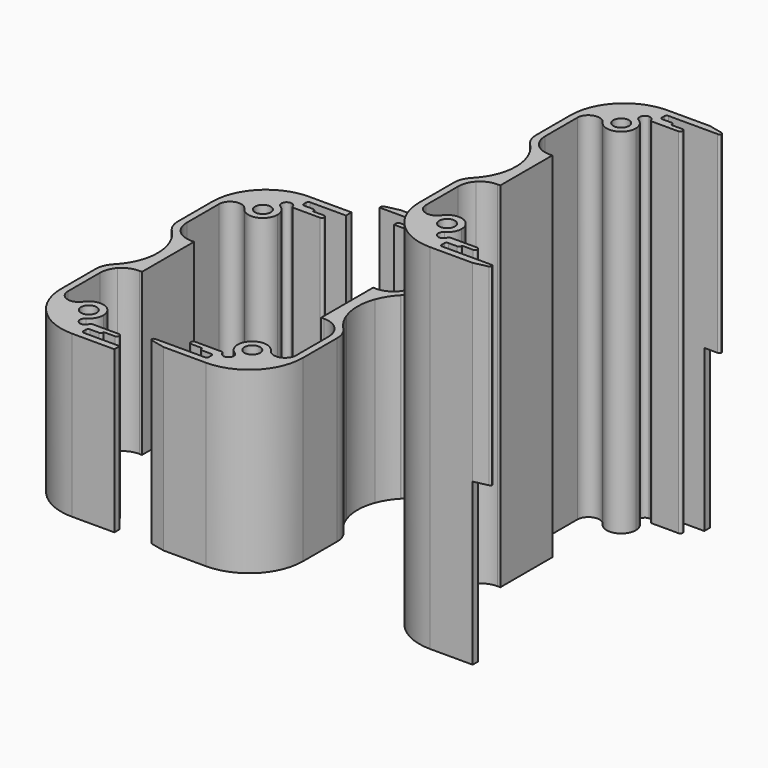
from build123d import *

# Parameters (mm, degrees)
F0_R          = 1.75
F0_W          = 4.8
F0_H          = 1.5477275198
F1_DEPTH      = 79
F2_DEPTH      = 40
F3_DEPTH      = 36
F4_T1_DEPTH   = 79
F4_T3_DEPTH   = 90.2941924891
F4_2_T1_DEPTH = 40
F4_2_T3_DEPTH = 51.2941924891
F4_3_T1_DEPTH = 36
F4_3_T3_DEPTH = 47.2941924891
F5_T1_DEPTH   = 79
F5_T3_DEPTH   = 81.0076197192
F5_T5_DEPTH   = 81.5
F5_T7_DEPTH   = 81.1160384943
F5_2_T1_DEPTH = 40
F5_2_T3_DEPTH = 42.0076197192
F5_2_T5_DEPTH = 42.5
F5_2_T7_DEPTH = 42.1160384943
F5_3_F1_R     = 0.5
F5_3_F2_R     = 0.4999
F5_3_F3_R     = 0.5
F5_3_F4_R     = 0.4999
F5_3_F5_R     = 0.5
F5_3_F6_R     = 0.5
F5_3_F7_R     = 0.5
F5_3_F8_R     = 0.5
F5_3_F9_R     = 0.5
F5_3_F10_R    = 0.5
F5_3_F11_R    = 0.5
F5_3_F12_R    = 0.5
F5_3_F13_R    = 0.5
F5_3_F14_R    = 0.5
F5_3_F15_R    = 0.5
F5_3_F16_R    = 0.5
F6_W          = 6
F6_H          = 66.2
F7_DEPTH      = 79.001
F8_W          = 6
F8_H          = 66.2
F9_DEPTH      = 36


# Not quite as in the source:
# - a fillet or chamfer that OpenCascade refuses, or shapes differently, is made with other operations: its cross-section is extruded or revolved along the edge and cut away or added
# - a fillet or chamfer is up to 0.001 mm smaller than in the source, because OpenCascade refuses the exact size


with BuildPart() as f1:
    # F0 (on Top) → F1 (new body)
    with BuildSketch(Plane.XY):
        with BuildLine():
            Line((-7, 11.0797111876), (-7, 9.2741576437))
            ThreePointArc((-7, 9.2741576437), (-6.2214566954, 8.6496058512), (-5.5, 7.9598994969))
            Line((-5.5, 7.9598994969), (-5.5, 10.0054984883))
            ThreePointArc((-5.5, 10.0054984883), (-6.2309192612, 10.5692486379), (-7, 11.0797111876))
        make_face()
        with BuildLine():
            ThreePointArc((-5.5, 21.1), (-2.7701351338, 28.1622234461), (4.0000000006, 31.5522724802))
            Line((4.0000000006, 31.5522724802), (4.0000000006, 33.0582607432))
            ThreePointArc((4.0000000006, 33.0582607432), (-3.8317608661, 29.2240384049), (-7, 21.1))
            Line((-7, 21.1), (-7, 11.0797111876))
            ThreePointArc((-7, 11.0797111876), (-6.2309192612, 10.5692486379), (-5.5, 10.0054984883))
            Line((-5.5, 10.0054984883), (-5.5, 21.1))
        make_face()
        with BuildLine():
            Line((-5.5, 10.0054984883), (-5.5, 7.9598994969))
            ThreePointArc((-5.5, 7.9598994969), (-4.0491111778, 6.0967341403), (-3.0093790725, 3.9764934301))
            Line((-3.0093790725, 3.9764934301), (-3.0093790725, 7.25))
            ThreePointArc((-3.0093790725, 7.25), (-4.1557714239, 8.7171586639), (-5.5, 10.0054984883))
        make_face()
        with BuildLine():
            Line((-3.0093790725, -3.9764934301), (-3.0093790725, -7.25))
            ThreePointArc((-3.0093790725, -7.25), (-1.3646055138, -3.7895862533), (-0.8, 0))
            ThreePointArc((-0.8, 0), (-1.3646055138, 3.7895862533), (-3.0093790725, 7.25))
            Line((-3.0093790725, 7.25), (-3.0093790725, 3.9764934301))
            ThreePointArc((-3.0093790725, 3.9764934301), (-2.4787337134, 2.0196360234), (-2.3, 0))
            ThreePointArc((-2.3, 0), (-2.4787337134, -2.0196360234), (-3.0093790725, -3.9764934301))
        make_face()
        with BuildLine():
            Line((-5.5, -7.9598994969), (-5.5, -10.0054984883))
            ThreePointArc((-5.5, -10.0054984883), (-4.1557714239, -8.7171586639), (-3.0093790725, -7.25))
            Line((-3.0093790725, -7.25), (-3.0093790725, -3.9764934301))
            ThreePointArc((-3.0093790725, -3.9764934301), (-4.0491111778, -6.0967341403), (-5.5, -7.9598994969))
        make_face()
        with BuildLine():
            Line((-7, -9.2741576437), (-7, -11.0797111876))
            ThreePointArc((-7, -11.0797111876), (-6.2309192612, -10.5692486379), (-5.5, -10.0054984883))
            Line((-5.5, -10.0054984883), (-5.5, -7.9598994969))
            ThreePointArc((-5.5, -7.9598994969), (-6.2214566954, -8.6496058512), (-7, -9.2741576437))
        make_face()
        with BuildLine():
            Line((5, -33.1), (6.0000000006, -33.1))
            Line((6.0000000006, -33.1), (6.0000000006, -31.6))
            Line((6.0000000006, -31.6), (5, -31.6))
            ThreePointArc((5, -31.6), (4.4994308452, -31.5880613328), (4.0000000006, -31.5522724802))
            ThreePointArc((4.0000000006, -31.5522724802), (-2.7701351338, -28.1622234461), (-5.5, -21.1))
            Line((-5.5, -21.1), (-5.5, -10.0054984883))
            ThreePointArc((-5.5, -10.0054984883), (-6.2309192612, -10.5692486379), (-7, -11.0797111876))
            Line((-7, -11.0797111876), (-7, -21.1))
            ThreePointArc((-7, -21.1), (-3.4852813742, -29.5852813742), (5, -33.1))
        make_face()
        with BuildLine():
            ThreePointArc((-5.5, -21.1), (-2.7701351338, -28.1622234461), (4.0000000006, -31.5522724802))
            Line((4.0000000006, -31.5522724802), (4.0000000006, -29.2661634937))
            ThreePointArc((4.0000000006, -29.2661634937), (2.875248939, -28.408013544), (3.4058490733, -27.0965449838))
            ThreePointArc((3.4058490733, -27.0965449838), (-0.6127011239, -26.5316234895), (-0.9475889999, -22.4874014267))
            ThreePointArc((-0.9475889999, -22.4874014267), (-3.7375818679, -23.4795655398), (-5.5, -21.1))
        make_face()
        with BuildLine():
            ThreePointArc((5, -24.3), (2.6974533631, -21.1911686883), (-0.9475889999, -22.4874014267))
            ThreePointArc((-0.9475889999, -22.4874014267), (-0.6127011239, -26.5316234895), (3.4058490733, -27.0965449838))
            ThreePointArc((3.4058490733, -27.0965449838), (4.5734738788, -25.9095015551), (5, -24.3))
        make_face()
        with Locations((1.75, -24.3)):
            Circle(F0_R, mode=Mode.SUBTRACT)
        with BuildLine():
            Line((5, -31.6), (6.0000000006, -31.6))
            Line((6.0000000006, -31.6), (6.0000000006, -29.9))
            Line((6.0000000006, -29.9), (9.0000000006, -29.9))
            Line((9.0000000006, -29.9), (9.0000000006, -29.2))
            Line((9.0000000006, -29.2), (12.0000000006, -29.2))
            Line((12.0000000006, -29.2), (12.0000000006, -28.1))
            Line((12.0000000006, -28.1), (5.1661634942, -28.1))
            ThreePointArc((5.1661634942, -28.1), (4.8246021149, -28.9246021143), (4.0000000006, -29.2661634937))
            Line((4.0000000006, -29.2661634937), (4.0000000006, -31.5522724802))
            ThreePointArc((4.0000000006, -31.5522724802), (4.4994308452, -31.5880613328), (5, -31.6))
        make_face()
        Polygon((6.0000000006, -33.1), (14.5, -33.1), (18, -32.3261362401), (18, -31.6), (6.0000000006, -31.6), align=None)
        with BuildLine():
            Line((4.0000000006, 29.2661634937), (4.0000000006, 31.5522724802))
            ThreePointArc((4.0000000006, 31.5522724802), (-2.7701351338, 28.1622234461), (-5.5, 21.1))
            ThreePointArc((-5.5, 21.1), (-3.7375818642, 23.4795655409), (-0.9475889956, 22.4874014203))
            ThreePointArc((-0.9475889956, 22.4874014203), (-0.612701148, 26.531623464), (3.4058490196, 27.0965450156))
            ThreePointArc((3.4058490196, 27.0965450156), (2.8752489472, 28.408013574), (4.0000000006, 29.2661634937))
        make_face()
        with BuildLine():
            ThreePointArc((3.4058490196, 27.0965450156), (-0.612701148, 26.531623464), (-0.9475889956, 22.4874014203))
            ThreePointArc((-0.9475889956, 22.4874014203), (2.6974533668, 21.1911686894), (5, 24.3))
            ThreePointArc((5, 24.3), (4.5734738633, 25.9095015822), (3.4058490196, 27.0965450156))
        make_face()
        with Locations((1.75, 24.3)):
            Circle(F0_R, mode=Mode.SUBTRACT)
        with BuildLine():
            Line((6.0000000006, 29.9), (6.0000000006, 31.5522724802))
            Line((6.0000000006, 31.5522724802), (4.0000000006, 31.5522724802))
            Line((4.0000000006, 31.5522724802), (4.0000000006, 29.2661634937))
            ThreePointArc((4.0000000006, 29.2661634937), (4.8246021149, 28.9246021143), (5.1661634942, 28.1))
            Line((5.1661634942, 28.1), (12.0000000006, 28.1))
            Line((12.0000000006, 28.1), (12.0000000006, 29.2))
            Line((12.0000000006, 29.2), (9.0000000006, 29.2))
            Line((9.0000000006, 29.2), (9.0000000006, 29.9))
            Line((9.0000000006, 29.9), (6.0000000006, 29.9))
        make_face()
        with Locations((8.4000000006, 32.3261362401)):
            Rectangle(F0_W, F0_H)
        Polygon((10.8000000006, 31.5522724802), (18, 31.5522724802), (18, 32.3261362401), (14.5, 33.1), (10.8000000006, 33.1), align=None)
        with BuildLine():
            Line((4.0000000006, 31.5522724802), (6.0000000006, 31.5522724802))
            Line((6.0000000006, 31.5522724802), (6.0000000006, 33.1))
            Line((6.0000000006, 33.1), (5, 33.1))
            ThreePointArc((5, 33.1), (4.4995646484, 33.0895606449), (4.0000000006, 33.0582607432))
            Line((4.0000000006, 33.0582607432), (4.0000000006, 31.5522724802))
        make_face()
        with BuildLine():
            ThreePointArc((-0.8, 0), (-1.3646055138, -3.7895862533), (-3.0093790725, -7.25))
            Line((-3.0093790725, -7.25), (0, -7.25))
            Line((0, -7.25), (0, 7.25))
            Line((0, 7.25), (-3.0093790725, 7.25))
            ThreePointArc((-3.0093790725, 7.25), (-1.3646055138, 3.7895862533), (-0.8, 0))
        make_face()
    extrude(amount=F1_DEPTH)

    # F4: fillet of radius 5 on 6 edges, made by hand

    # F4_s2 → F4_t1 (join)
    with BuildSketch(Plane.XY):
        with BuildLine():
            ThreePointArc((-5.5, -12.1288911282), (-5.1622002436, -10.3222675125), (-4.1944444444, -8.7597547037))
            ThreePointArc((-4.1944444444, -8.7597547037), (-4.8255808359, -9.405307048), (-5.5, -10.0054984883))
            Line((-5.5, -10.0054984883), (-5.5, -12.1288911282))
        make_face()
        with BuildLine():
            ThreePointArc((-4.2749457245, -8.8472222222), (-2.6097264456, -7.6666666667), (-0.6114633109, -7.25))
            Line((-0.6114633109, -7.25), (-3.0093790725, -7.25))
            ThreePointArc((-3.0093790725, -7.25), (-3.6108172828, -8.0734475632), (-4.2749457245, -8.8472222222))
        make_face()
        with BuildLine():
            ThreePointArc((-4.1944444444, 8.7597547037), (-5.1622002436, 10.3222675125), (-5.5, 12.1288911282))
            Line((-5.5, 12.1288911282), (-5.5, 10.0054984883))
            ThreePointArc((-5.5, 10.0054984883), (-4.8255808359, 9.405307048), (-4.1944444444, 8.7597547037))
        make_face()
        with BuildLine():
            ThreePointArc((-0.6114633109, 7.25), (-2.6097264456, 7.6666666667), (-4.2749457245, 8.8472222222))
            ThreePointArc((-4.2749457245, 8.8472222222), (-3.6108172828, 8.0734475632), (-3.0093790725, 7.25))
            Line((-3.0093790725, 7.25), (-0.6114633109, 7.25))
        make_face()
    extrude(amount=F4_T1_DEPTH)

    # F4_s4 → F4_t3 (cut)
    with BuildSketch(Plane.XY.offset(-5.6470962445)):
        with BuildLine():
            ThreePointArc((-5.5757575758, 8.0381488259), (-6.6302693161, 9.6460393162), (-7, 11.5329961415))
            Line((-7, 11.5329961415), (-7, 9.2741576437))
            ThreePointArc((-7, 9.2741576437), (-6.2625007758, 8.6853961018), (-5.5757575758, 8.0381488259))
        make_face()
        with BuildLine():
            ThreePointArc((-5.5757575758, -8.0381488259), (-6.6302693161, -9.6460393162), (-7, -11.5329961415))
            Line((-7, -11.5329961415), (-7, -9.2741576437))
            ThreePointArc((-7, -9.2741576437), (-6.2625007758, -8.6853961018), (-5.5757575758, -8.0381488259))
        make_face()
    extrude(amount=F4_T3_DEPTH, mode=Mode.SUBTRACT)

    # F5: fillet of radius 0.5 on 16 edges, made by hand

    # F5_s2 → F5_t1 (join)
    with BuildSketch(Plane.XY):
        with BuildLine():
            ThreePointArc((6.5000000006, -29.9), (6.14644661, -30.0464466094), (6.0000000006, -30.4))
            Line((6.0000000006, -30.4), (6.0000000006, -29.9))
            Line((6.0000000006, -29.9), (6.5000000006, -29.9))
        make_face()
        with BuildLine():
            ThreePointArc((6.0000000006, -31.1), (6.14644661, -31.4535533906), (6.5000000006, -31.6))
            Line((6.5000000006, -31.6), (6.0000000006, -31.6))
            Line((6.0000000006, -31.6), (6.0000000006, -31.1))
        make_face()
        with BuildLine():
            ThreePointArc((6.5000000006, 31.5522724802), (6.14644661, 31.4058258708), (6.0000000006, 31.0522724802))
            Line((6.0000000006, 31.0522724802), (6.0000000006, 31.5522724802))
            Line((6.0000000006, 31.5522724802), (6.5000000006, 31.5522724802))
        make_face()
        with BuildLine():
            ThreePointArc((6.0000000006, 30.4), (6.14644661, 30.0464466094), (6.5000000006, 29.9))
            Line((6.5000000006, 29.9), (6.0000000006, 29.9))
            Line((6.0000000006, 29.9), (6.0000000006, 30.4))
        make_face()
    extrude(amount=F5_T1_DEPTH)

    # F5_s4 → F5_t3 (cut)
    with BuildSketch(Plane.XY.offset(-1.0038098596)):
        with BuildLine():
            ThreePointArc((18, -31.9246122963), (17.8898541073, -32.2376838137), (17.6079449, -32.4128211641))
            Line((17.6079449, -32.4128211641), (18, -32.3261362401))
            Line((18, -32.3261362401), (18, -31.9246122963))
        make_face()
        with BuildLine():
            ThreePointArc((17.6079449, 32.4128211641), (17.8898541073, 32.2376838137), (18, 31.9246122963))
            Line((18, 31.9246122963), (18, 32.3261362401))
            Line((18, 32.3261362401), (17.6079449, 32.4128211641))
        make_face()
    extrude(amount=F5_T3_DEPTH, mode=Mode.SUBTRACT)

    # F5_s6 → F5_t5 (cut)
    with BuildSketch(Plane.XY.offset(-1.25)):
        with BuildLine():
            ThreePointArc((17.5, -31.6), (17.8535533906, -31.7464466094), (18, -32.1))
            Line((18, -32.1), (18, -31.6))
            Line((18, -31.6), (17.5, -31.6))
        make_face()
        with BuildLine():
            ThreePointArc((9.0000000006, -29.4), (8.8535533912, -29.7535533906), (8.5000000006, -29.9))
            Line((8.5000000006, -29.9), (9.0000000006, -29.9))
            Line((9.0000000006, -29.9), (9.0000000006, -29.4))
        make_face()
        with BuildLine():
            ThreePointArc((12.0000000006, -28.7), (11.8535533912, -29.0535533906), (11.5000000006, -29.2))
            Line((11.5000000006, -29.2), (12.0000000006, -29.2))
            Line((12.0000000006, -29.2), (12.0000000006, -28.7))
        make_face()
        with BuildLine():
            ThreePointArc((11.5000000006, -28.1), (11.8535533912, -28.2464466094), (12.0000000006, -28.6))
            Line((12.0000000006, -28.6), (12.0000000006, -28.1))
            Line((12.0000000006, -28.1), (11.5000000006, -28.1))
        make_face()
        with BuildLine():
            ThreePointArc((18, 32.0522724802), (17.8535533906, 31.6987190896), (17.5, 31.5522724802))
            Line((17.5, 31.5522724802), (18, 31.5522724802))
            Line((18, 31.5522724802), (18, 32.0522724802))
        make_face()
        with BuildLine():
            ThreePointArc((8.5000000006, 29.9), (8.8535533912, 29.7535533906), (9.0000000006, 29.4))
            Line((9.0000000006, 29.4), (9.0000000006, 29.9))
            Line((9.0000000006, 29.9), (8.5000000006, 29.9))
        make_face()
        with BuildLine():
            ThreePointArc((12.0000000006, 28.6), (11.8535533912, 28.2464466094), (11.5000000006, 28.1))
            Line((11.5000000006, 28.1), (12.0000000006, 28.1))
            Line((12.0000000006, 28.1), (12.0000000006, 28.6))
        make_face()
        with BuildLine():
            ThreePointArc((11.5000000006, 29.2), (11.8535533912, 29.0535533906), (12.0000000006, 28.7))
            Line((12.0000000006, 28.7), (12.0000000006, 29.2))
            Line((12.0000000006, 29.2), (11.5000000006, 29.2))
        make_face()
    extrude(amount=F5_T5_DEPTH, mode=Mode.SUBTRACT)

    # F5_s8 → F5_t7 (cut)
    with BuildSketch(Plane.XY.offset(-1.0580192471)):
        with BuildLine():
            ThreePointArc((5.1124158407, -28.4499547008), (5.293586347, -28.1968730661), (5.5893711931, -28.1))
            Line((5.5893711931, -28.1), (5.1661634942, -28.1))
            ThreePointArc((5.1661634942, -28.1), (5.1526482636, -28.277029025), (5.1124158407, -28.4499547008))
        make_face()
        with BuildLine():
            ThreePointArc((5.5893711931, 28.1), (5.293586347, 28.1968730661), (5.1124158407, 28.4499547008))
            ThreePointArc((5.1124158407, 28.4499547008), (5.1526482636, 28.277029025), (5.1661634942, 28.1))
            Line((5.1661634942, 28.1), (5.5893711931, 28.1))
        make_face()
    extrude(amount=F5_T7_DEPTH, mode=Mode.SUBTRACT)

    # F8 (on face) → F9 (cut)
    with BuildSketch(Plane(origin=(0, 0, 0), x_dir=(1, 0, 0), z_dir=(0, 0, -1))):
        with Locations((17.5, 0)):
            Rectangle(F8_W, F8_H)
    extrude(amount=-F9_DEPTH, mode=Mode.SUBTRACT)


with BuildPart() as f2:
    # F0 (on Top) → F2 (new body)
    with BuildSketch(Plane.XY):
        with BuildLine():
            ThreePointArc((-34.5, 10.0054984883), (-33.7690807388, 10.5692486379), (-33, 11.0797111876))
            Line((-33, 11.0797111876), (-33, 21.1))
            ThreePointArc((-33, 21.1), (-36.1682391339, 29.2240384049), (-44.0000000006, 33.0582607432))
            Line((-44.0000000006, 33.0582607432), (-44.0000000006, 31.5522724802))
            ThreePointArc((-44.0000000006, 31.5522724802), (-37.2298648662, 28.1622234461), (-34.5, 21.1))
            Line((-34.5, 21.1), (-34.5, 10.0054984883))
        make_face()
        Polygon((-54.5, -33.1), (-46.0000000006, -33.1), (-46.0000000006, -31.6), (-58, -31.6), (-58, -32.3261362401), align=None)
        with BuildLine():
            Line((-33, -21.1), (-33, -11.0797111876))
            ThreePointArc((-33, -11.0797111876), (-33.7690807388, -10.5692486379), (-34.5, -10.0054984883))
            Line((-34.5, -10.0054984883), (-34.5, -21.1))
            ThreePointArc((-34.5, -21.1), (-37.2298648662, -28.1622234461), (-44.0000000006, -31.5522724802))
            ThreePointArc((-44.0000000006, -31.5522724802), (-44.4994308452, -31.5880613328), (-45, -31.6))
            Line((-45, -31.6), (-46.0000000006, -31.6))
            Line((-46.0000000006, -31.6), (-46.0000000006, -33.1))
            Line((-46.0000000006, -33.1), (-45, -33.1))
            ThreePointArc((-45, -33.1), (-36.5147186258, -29.5852813742), (-33, -21.1))
        make_face()
        with BuildLine():
            ThreePointArc((-45, -31.6), (-44.4994308452, -31.5880613328), (-44.0000000006, -31.5522724802))
            Line((-44.0000000006, -31.5522724802), (-44.0000000006, -29.2661634937))
            ThreePointArc((-44.0000000006, -29.2661634937), (-44.8246021149, -28.9246021143), (-45.1661634942, -28.1))
            Line((-45.1661634942, -28.1), (-52.0000000006, -28.1))
            Line((-52.0000000006, -28.1), (-52.0000000006, -29.2))
            Line((-52.0000000006, -29.2), (-49.0000000006, -29.2))
            Line((-49.0000000006, -29.2), (-49.0000000006, -29.9))
            Line((-49.0000000006, -29.9), (-46.0000000006, -29.9))
            Line((-46.0000000006, -29.9), (-46.0000000006, -31.6))
            Line((-46.0000000006, -31.6), (-45, -31.6))
        make_face()
        with BuildLine():
            ThreePointArc((-44.0000000006, -31.5522724802), (-37.2298648662, -28.1622234461), (-34.5, -21.1))
            ThreePointArc((-34.5, -21.1), (-36.2624181353, -23.4795655408), (-39.0524110039, -22.4874014212))
            ThreePointArc((-39.0524110039, -22.4874014212), (-38.6411686893, -23.3525466337), (-38.5, -24.3))
            ThreePointArc((-38.5, -24.3), (-40.1404982423, -27.1234737633), (-43.4058486719, -27.0965452215))
            ThreePointArc((-43.4058486719, -27.0965452215), (-42.9868823166, -27.5224795654), (-42.8338365069, -28.1))
            ThreePointArc((-42.8338365069, -28.1), (-43.1753978863, -28.9246021143), (-44.0000000006, -29.2661634937))
            Line((-44.0000000006, -29.2661634937), (-44.0000000006, -31.5522724802))
        make_face()
        with BuildLine():
            ThreePointArc((-38.5, -24.3), (-38.6411686893, -23.3525466337), (-39.0524110039, -22.4874014212))
            ThreePointArc((-39.0524110039, -22.4874014212), (-44.1127012864, -22.0683766825), (-43.4058486719, -27.0965452215))
            ThreePointArc((-43.4058486719, -27.0965452215), (-40.1404982423, -27.1234737633), (-38.5, -24.3))
        make_face()
        with Locations((-41.75, -24.3)):
            Circle(F0_R, mode=Mode.SUBTRACT)
        with BuildLine():
            ThreePointArc((-34.5, -10.0054984883), (-33.7690807388, -10.5692486379), (-33, -11.0797111876))
            Line((-33, -11.0797111876), (-33, -9.2741576437))
            ThreePointArc((-33, -9.2741576437), (-33.7785433046, -8.6496058512), (-34.5, -7.9598994969))
            Line((-34.5, -7.9598994969), (-34.5, -10.0054984883))
        make_face()
        with BuildLine():
            ThreePointArc((-36.9906209275, -7.25), (-35.8442285761, -8.7171586639), (-34.5, -10.0054984883))
            Line((-34.5, -10.0054984883), (-34.5, -7.9598994969))
            ThreePointArc((-34.5, -7.9598994969), (-35.9508888222, -6.0967341403), (-36.9906209275, -3.9764934301))
            Line((-36.9906209275, -3.9764934301), (-36.9906209275, -7.25))
        make_face()
        with BuildLine():
            Line((-40, -7.25), (-36.9906209275, -7.25))
            ThreePointArc((-36.9906209275, -7.25), (-39.2, 0), (-36.9906209275, 7.25))
            Line((-36.9906209275, 7.25), (-40, 7.25))
            Line((-40, 7.25), (-40, -7.25))
        make_face()
        with BuildLine():
            ThreePointArc((-36.9906209275, 7.25), (-39.2, 0), (-36.9906209275, -7.25))
            Line((-36.9906209275, -7.25), (-36.9906209275, -3.9764934301))
            ThreePointArc((-36.9906209275, -3.9764934301), (-37.7, 0), (-36.9906209275, 3.9764934301))
            Line((-36.9906209275, 3.9764934301), (-36.9906209275, 7.25))
        make_face()
        with BuildLine():
            ThreePointArc((-36.9906209275, 3.9764934301), (-35.9508888222, 6.0967341403), (-34.5, 7.9598994969))
            Line((-34.5, 7.9598994969), (-34.5, 10.0054984883))
            ThreePointArc((-34.5, 10.0054984883), (-35.8442285761, 8.7171586639), (-36.9906209275, 7.25))
            Line((-36.9906209275, 7.25), (-36.9906209275, 3.9764934301))
        make_face()
        with BuildLine():
            ThreePointArc((-34.5, 7.9598994969), (-33.7785433046, 8.6496058512), (-33, 9.2741576437))
            Line((-33, 9.2741576437), (-33, 11.0797111876))
            ThreePointArc((-33, 11.0797111876), (-33.7690807388, 10.5692486379), (-34.5, 10.0054984883))
            Line((-34.5, 10.0054984883), (-34.5, 7.9598994969))
        make_face()
        with BuildLine():
            ThreePointArc((-39.0524110298, 22.4874013826), (-36.2624181576, 23.4795655476), (-34.5, 21.1))
            ThreePointArc((-34.5, 21.1), (-37.2298648662, 28.1622234461), (-44.0000000006, 31.5522724802))
            Line((-44.0000000006, 31.5522724802), (-44.0000000006, 29.2661634937))
            ThreePointArc((-44.0000000006, 29.2661634937), (-43.1753978863, 28.9246021143), (-42.8338365069, 28.1))
            ThreePointArc((-42.8338365069, 28.1), (-42.9868823175, 27.5224795638), (-43.4058486751, 27.0965452196))
            ThreePointArc((-43.4058486751, 27.0965452196), (-40.1404982439, 27.1234737642), (-38.5, 24.3))
            ThreePointArc((-38.5, 24.3), (-38.641168696, 23.3525466115), (-39.0524110298, 22.4874013826))
        make_face()
        with BuildLine():
            ThreePointArc((-43.4058486751, 27.0965452196), (-44.1127013011, 22.068376698), (-39.0524110298, 22.4874013826))
            ThreePointArc((-39.0524110298, 22.4874013826), (-38.641168696, 23.3525466115), (-38.5, 24.3))
            ThreePointArc((-38.5, 24.3), (-40.1404982439, 27.1234737642), (-43.4058486751, 27.0965452196))
        make_face()
        with Locations((-41.75, 24.3)):
            Circle(F0_R, mode=Mode.SUBTRACT)
        with BuildLine():
            Line((-44.0000000006, 29.2661634937), (-44.0000000006, 31.5522724802))
            Line((-44.0000000006, 31.5522724802), (-46.0000000006, 31.5522724802))
            Line((-46.0000000006, 31.5522724802), (-46.0000000006, 29.9))
            Line((-46.0000000006, 29.9), (-49.0000000006, 29.9))
            Line((-49.0000000006, 29.9), (-49.0000000006, 29.2))
            Line((-49.0000000006, 29.2), (-52.0000000006, 29.2))
            Line((-52.0000000006, 29.2), (-52.0000000006, 28.1))
            Line((-52.0000000006, 28.1), (-45.1661634942, 28.1))
            ThreePointArc((-45.1661634942, 28.1), (-44.8246021149, 28.9246021143), (-44.0000000006, 29.2661634937))
        make_face()
        with Locations((-48.4000000006, 32.3261362401)):
            Rectangle(F0_W, F0_H)
        Polygon((-58, 32.3261362401), (-58, 31.5522724802), (-50.8000000006, 31.5522724802), (-50.8000000006, 33.1), (-54.5, 33.1), align=None)
        with BuildLine():
            Line((-44.0000000006, 31.5522724802), (-44.0000000006, 33.0582607432))
            ThreePointArc((-44.0000000006, 33.0582607432), (-44.4995646484, 33.0895606449), (-45, 33.1))
            Line((-45, 33.1), (-46.0000000006, 33.1))
            Line((-46.0000000006, 33.1), (-46.0000000006, 31.5522724802))
            Line((-46.0000000006, 31.5522724802), (-44.0000000006, 31.5522724802))
        make_face()
    extrude(amount=F2_DEPTH)

    # F4#2: fillet of radius 5 on 6 edges, made by hand

    # F4_2_s2 → F4_2_t1 (join)
    with BuildSketch(Plane.XY):
        with BuildLine():
            ThreePointArc((-34.5, 12.1288911282), (-34.8377997564, 10.3222675125), (-35.8055555556, 8.7597547037))
            ThreePointArc((-35.8055555556, 8.7597547037), (-35.1744191641, 9.405307048), (-34.5, 10.0054984883))
            Line((-34.5, 10.0054984883), (-34.5, 12.1288911282))
        make_face()
        with BuildLine():
            ThreePointArc((-35.8055555556, -8.7597547037), (-34.8377997564, -10.3222675125), (-34.5, -12.1288911282))
            Line((-34.5, -12.1288911282), (-34.5, -10.0054984883))
            ThreePointArc((-34.5, -10.0054984883), (-35.1744191641, -9.405307048), (-35.8055555556, -8.7597547037))
        make_face()
        with BuildLine():
            ThreePointArc((-39.3885366891, -7.25), (-37.3902735544, -7.6666666667), (-35.7250542755, -8.8472222222))
            ThreePointArc((-35.7250542755, -8.8472222222), (-36.3891827172, -8.0734475632), (-36.9906209275, -7.25))
            Line((-36.9906209275, -7.25), (-39.3885366891, -7.25))
        make_face()
        with BuildLine():
            ThreePointArc((-35.7250542755, 8.8472222222), (-37.3902735544, 7.6666666667), (-39.3885366891, 7.25))
            Line((-39.3885366891, 7.25), (-36.9906209275, 7.25))
            ThreePointArc((-36.9906209275, 7.25), (-36.3891827172, 8.0734475632), (-35.7250542755, 8.8472222222))
        make_face()
    extrude(amount=F4_2_T1_DEPTH)

    # F4_2_s4 → F4_2_t3 (cut)
    with BuildSketch(Plane.XY.offset(-5.6470962445)):
        with BuildLine():
            ThreePointArc((-34.4242424242, -8.0381488259), (-33.3697306839, -9.6460393162), (-33, -11.5329961415))
            Line((-33, -11.5329961415), (-33, -9.2741576437))
            ThreePointArc((-33, -9.2741576437), (-33.7374992242, -8.6853961018), (-34.4242424242, -8.0381488259))
        make_face()
        with BuildLine():
            ThreePointArc((-33, 11.5329961415), (-33.3697306839, 9.6460393162), (-34.4242424242, 8.0381488259))
            ThreePointArc((-34.4242424242, 8.0381488259), (-33.7374992242, 8.6853961018), (-33, 9.2741576437))
            Line((-33, 9.2741576437), (-33, 11.5329961415))
        make_face()
    extrude(amount=F4_2_T3_DEPTH, mode=Mode.SUBTRACT)

    # F5#2: fillet of radius 0.5 on 14 edges, made by hand

    # F5_2_s2 → F5_2_t1 (join)
    with BuildSketch(Plane.XY):
        with BuildLine():
            ThreePointArc((-46.0000000006, 31.0522724802), (-46.14644661, 31.4058258708), (-46.5000000006, 31.5522724802))
            Line((-46.5000000006, 31.5522724802), (-46.0000000006, 31.5522724802))
            Line((-46.0000000006, 31.5522724802), (-46.0000000006, 31.0522724802))
        make_face()
        with BuildLine():
            ThreePointArc((-46.5000000006, 29.9), (-46.14644661, 30.0464466094), (-46.0000000006, 30.4))
            Line((-46.0000000006, 30.4), (-46.0000000006, 29.9))
            Line((-46.0000000006, 29.9), (-46.5000000006, 29.9))
        make_face()
        with BuildLine():
            ThreePointArc((-46.0000000006, -30.4), (-46.14644661, -30.0464466094), (-46.5000000006, -29.9))
            Line((-46.5000000006, -29.9), (-46.0000000006, -29.9))
            Line((-46.0000000006, -29.9), (-46.0000000006, -30.4))
        make_face()
        with BuildLine():
            ThreePointArc((-46.5000000006, -31.6), (-46.14644661, -31.4535533906), (-46.0000000006, -31.1))
            Line((-46.0000000006, -31.1), (-46.0000000006, -31.6))
            Line((-46.0000000006, -31.6), (-46.5000000006, -31.6))
        make_face()
    extrude(amount=F5_2_T1_DEPTH)

    # F5_2_s4 → F5_2_t3 (cut)
    with BuildSketch(Plane.XY.offset(-1.0038098596)):
        with BuildLine():
            ThreePointArc((-57.6079449, 32.4128211641), (-57.8898541073, 32.2376838137), (-58, 31.9246122963))
            Line((-58, 31.9246122963), (-58, 32.3261362401))
            Line((-58, 32.3261362401), (-57.6079449, 32.4128211641))
        make_face()
        with BuildLine():
            ThreePointArc((-57.6079449, -32.4128211641), (-57.8898541073, -32.2376838137), (-58, -31.9246122963))
            Line((-58, -31.9246122963), (-58, -32.3261362401))
            Line((-58, -32.3261362401), (-57.6079449, -32.4128211641))
        make_face()
    extrude(amount=F5_2_T3_DEPTH, mode=Mode.SUBTRACT)

    # F5_2_s6 → F5_2_t5 (cut)
    with BuildSketch(Plane.XY.offset(-1.25)):
        with BuildLine():
            ThreePointArc((-49.0000000006, 29.4), (-48.8535533912, 29.7535533906), (-48.5000000006, 29.9))
            Line((-48.5000000006, 29.9), (-49.0000000006, 29.9))
            Line((-49.0000000006, 29.9), (-49.0000000006, 29.4))
        make_face()
        with BuildLine():
            ThreePointArc((-52.0000000006, 28.7), (-51.8535533912, 29.0535533906), (-51.5000000006, 29.2))
            Line((-51.5000000006, 29.2), (-52.0000000006, 29.2))
            Line((-52.0000000006, 29.2), (-52.0000000006, 28.7))
        make_face()
        with BuildLine():
            ThreePointArc((-52.0000000006, -28.6), (-51.8535533912, -28.2464466094), (-51.5000000006, -28.1))
            Line((-51.5000000006, -28.1), (-52.0000000006, -28.1))
            Line((-52.0000000006, -28.1), (-52.0000000006, -28.6))
        make_face()
        with BuildLine():
            ThreePointArc((-51.5000000006, -29.2), (-51.8535533912, -29.0535533906), (-52.0000000006, -28.7))
            Line((-52.0000000006, -28.7), (-52.0000000006, -29.2))
            Line((-52.0000000006, -29.2), (-51.5000000006, -29.2))
        make_face()
        with BuildLine():
            ThreePointArc((-48.5000000006, -29.9), (-48.8535533912, -29.7535533906), (-49.0000000006, -29.4))
            Line((-49.0000000006, -29.4), (-49.0000000006, -29.9))
            Line((-49.0000000006, -29.9), (-48.5000000006, -29.9))
        make_face()
        with BuildLine():
            ThreePointArc((-58, -32.1), (-57.8535533906, -31.7464466094), (-57.5, -31.6))
            Line((-57.5, -31.6), (-58, -31.6))
            Line((-58, -31.6), (-58, -32.1))
        make_face()
    extrude(amount=F5_2_T5_DEPTH, mode=Mode.SUBTRACT)

    # F5_2_s8 → F5_2_t7 (cut)
    with BuildSketch(Plane.XY.offset(-1.0580192471)):
        with BuildLine():
            ThreePointArc((-45.1124158407, 28.4499547008), (-45.293586347, 28.1968730661), (-45.5893711931, 28.1))
            Line((-45.5893711931, 28.1), (-45.1661634942, 28.1))
            ThreePointArc((-45.1661634942, 28.1), (-45.1526482636, 28.277029025), (-45.1124158407, 28.4499547008))
        make_face()
        with BuildLine():
            ThreePointArc((-45.5893711931, -28.1), (-45.293586347, -28.1968730661), (-45.1124158407, -28.4499547008))
            ThreePointArc((-45.1124158407, -28.4499547008), (-45.1526482636, -28.277029025), (-45.1661634942, -28.1))
            Line((-45.1661634942, -28.1), (-45.5893711931, -28.1))
        make_face()
    extrude(amount=F5_2_T7_DEPTH, mode=Mode.SUBTRACT)


with BuildPart() as f3:
    # F0 (on Top) → F3 (new body)
    with BuildSketch(Plane.XY):
        with BuildLine():
            Line((-73.9999999994, -33.1), (-73.9999999994, -31.6))
            Line((-73.9999999994, -31.6), (-75, -31.6))
            ThreePointArc((-75, -31.6), (-75.5005691548, -31.5880613328), (-75.9999999994, -31.5522724802))
            ThreePointArc((-75.9999999994, -31.5522724802), (-82.7701351338, -28.1622234461), (-85.5, -21.1))
            Line((-85.5, -21.1), (-85.5, -10.0054984883))
            ThreePointArc((-85.5, -10.0054984883), (-86.2309192612, -10.5692486379), (-87, -11.0797111876))
            Line((-87, -11.0797111876), (-87, -21.1))
            ThreePointArc((-87, -21.1), (-83.4852813742, -29.5852813742), (-75, -33.1))
            Line((-75, -33.1), (-73.9999999994, -33.1))
        make_face()
        Polygon((-69.1999999994, 33.1), (-69.1999999994, 31.5522724802), (-62, 31.5522724802), (-62, 32.3261362401), (-65.5, 33.1), align=None)
        with Locations((-71.5999999994, 32.3261362401)):
            Rectangle(F0_W, F0_H)
        with BuildLine():
            Line((-75.9999999994, 33.0582607432), (-75.9999999994, 31.5522724802))
            Line((-75.9999999994, 31.5522724802), (-73.9999999994, 31.5522724802))
            Line((-73.9999999994, 31.5522724802), (-73.9999999994, 33.1))
            Line((-73.9999999994, 33.1), (-75, 33.1))
            ThreePointArc((-75, 33.1), (-75.5004353516, 33.0895606449), (-75.9999999994, 33.0582607432))
        make_face()
        with BuildLine():
            ThreePointArc((-75.9999999994, 29.2661634937), (-75.1753978851, 28.9246021143), (-74.8338365058, 28.1))
            Line((-74.8338365058, 28.1), (-67.9999999994, 28.1))
            Line((-67.9999999994, 28.1), (-67.9999999994, 29.2))
            Line((-67.9999999994, 29.2), (-70.9999999994, 29.2))
            Line((-70.9999999994, 29.2), (-70.9999999994, 29.9))
            Line((-70.9999999994, 29.9), (-73.9999999994, 29.9))
            Line((-73.9999999994, 29.9), (-73.9999999994, 31.5522724802))
            Line((-73.9999999994, 31.5522724802), (-75.9999999994, 31.5522724802))
            Line((-75.9999999994, 31.5522724802), (-75.9999999994, 29.2661634937))
        make_face()
        with BuildLine():
            ThreePointArc((-76.5941509639, 27.0965450058), (-77.1247510553, 28.4080135648), (-75.9999999994, 29.2661634937))
            Line((-75.9999999994, 29.2661634937), (-75.9999999994, 31.5522724802))
            ThreePointArc((-75.9999999994, 31.5522724802), (-82.7701351338, 28.1622234461), (-85.5, 21.1))
            ThreePointArc((-85.5, 21.1), (-83.7375816677, 23.4795656008), (-80.9475887664, 22.4874010793))
            ThreePointArc((-80.9475887664, 22.4874010793), (-80.6127012825, 26.5316233216), (-76.5941509639, 27.0965450058))
        make_face()
        with BuildLine():
            ThreePointArc((-75, 24.3), (-75.4265261319, 25.9095015739), (-76.5941509639, 27.0965450058))
            ThreePointArc((-76.5941509639, 27.0965450058), (-80.6127012825, 26.5316233216), (-80.9475887664, 22.4874010793))
            ThreePointArc((-80.9475887664, 22.4874010793), (-77.3025464367, 21.1911687493), (-75, 24.3))
        make_face()
        with Locations((-78.25, 24.3)):
            Circle(F0_R, mode=Mode.SUBTRACT)
        with BuildLine():
            ThreePointArc((-85.5, 21.1), (-82.7701351338, 28.1622234461), (-75.9999999994, 31.5522724802))
            Line((-75.9999999994, 31.5522724802), (-75.9999999994, 33.0582607432))
            ThreePointArc((-75.9999999994, 33.0582607432), (-83.8317608661, 29.2240384049), (-87, 21.1))
            Line((-87, 21.1), (-87, 11.0797111876))
            ThreePointArc((-87, 11.0797111876), (-86.2309192612, 10.5692486379), (-85.5, 10.0054984883))
            Line((-85.5, 10.0054984883), (-85.5, 21.1))
        make_face()
        with BuildLine():
            Line((-85.5, 7.9598994969), (-85.5, 10.0054984883))
            ThreePointArc((-85.5, 10.0054984883), (-86.2309192612, 10.5692486379), (-87, 11.0797111876))
            Line((-87, 11.0797111876), (-87, 9.2741576437))
            ThreePointArc((-87, 9.2741576437), (-86.2214566954, 8.6496058512), (-85.5, 7.9598994969))
        make_face()
        with BuildLine():
            ThreePointArc((-83.0093790725, 7.25), (-84.1557714239, 8.7171586639), (-85.5, 10.0054984883))
            Line((-85.5, 10.0054984883), (-85.5, 7.9598994969))
            ThreePointArc((-85.5, 7.9598994969), (-84.0491111778, 6.0967341403), (-83.0093790725, 3.9764934301))
            Line((-83.0093790725, 3.9764934301), (-83.0093790725, 7.25))
        make_face()
        with BuildLine():
            ThreePointArc((-80.8, 0), (-81.3646055138, 3.7895862533), (-83.0093790725, 7.25))
            Line((-83.0093790725, 7.25), (-83.0093790725, 3.9764934301))
            ThreePointArc((-83.0093790725, 3.9764934301), (-82.4787337134, 2.0196360234), (-82.3, 0))
            ThreePointArc((-82.3, 0), (-82.4787337134, -2.0196360234), (-83.0093790725, -3.9764934301))
            Line((-83.0093790725, -3.9764934301), (-83.0093790725, -7.25))
            ThreePointArc((-83.0093790725, -7.25), (-81.3646055138, -3.7895862533), (-80.8, 0))
        make_face()
        with BuildLine():
            Line((-80, 7.25), (-83.0093790725, 7.25))
            ThreePointArc((-83.0093790725, 7.25), (-81.3646055138, 3.7895862533), (-80.8, 0))
            ThreePointArc((-80.8, 0), (-81.3646055138, -3.7895862533), (-83.0093790725, -7.25))
            Line((-83.0093790725, -7.25), (-80, -7.25))
            Line((-80, -7.25), (-80, 7.25))
        make_face()
        with BuildLine():
            ThreePointArc((-83.0093790725, -3.9764934301), (-84.0491111778, -6.0967341403), (-85.5, -7.9598994969))
            Line((-85.5, -7.9598994969), (-85.5, -10.0054984883))
            ThreePointArc((-85.5, -10.0054984883), (-84.1557714239, -8.7171586639), (-83.0093790725, -7.25))
            Line((-83.0093790725, -7.25), (-83.0093790725, -3.9764934301))
        make_face()
        with BuildLine():
            Line((-85.5, -10.0054984883), (-85.5, -7.9598994969))
            ThreePointArc((-85.5, -7.9598994969), (-86.2214566954, -8.6496058512), (-87, -9.2741576437))
            Line((-87, -9.2741576437), (-87, -11.0797111876))
            ThreePointArc((-87, -11.0797111876), (-86.2309192612, -10.5692486379), (-85.5, -10.0054984883))
        make_face()
        with BuildLine():
            ThreePointArc((-80.9475887664, -22.4874010793), (-83.7375816677, -23.4795656008), (-85.5, -21.1))
            ThreePointArc((-85.5, -21.1), (-82.7701351338, -28.1622234461), (-75.9999999994, -31.5522724802))
            Line((-75.9999999994, -31.5522724802), (-75.9999999994, -29.2661634937))
            ThreePointArc((-75.9999999994, -29.2661634937), (-77.1247510466, -28.4080135968), (-76.594151021, -27.0965450396))
            ThreePointArc((-76.594151021, -27.0965450396), (-80.6127013053, -26.5316232975), (-80.9475887664, -22.4874010793))
        make_face()
        with BuildLine():
            ThreePointArc((-75, -24.3), (-77.3025464367, -21.1911687493), (-80.9475887664, -22.4874010793))
            ThreePointArc((-80.9475887664, -22.4874010793), (-80.6127013053, -26.5316232975), (-76.594151021, -27.0965450396))
            ThreePointArc((-76.594151021, -27.0965450396), (-75.4265261484, -25.9095016027), (-75, -24.3))
        make_face()
        with Locations((-78.25, -24.3)):
            Circle(F0_R, mode=Mode.SUBTRACT)
        with BuildLine():
            Line((-75, -31.6), (-73.9999999994, -31.6))
            Line((-73.9999999994, -31.6), (-73.9999999994, -29.9))
            Line((-73.9999999994, -29.9), (-70.9999999994, -29.9))
            Line((-70.9999999994, -29.9), (-70.9999999994, -29.2))
            Line((-70.9999999994, -29.2), (-67.9999999994, -29.2))
            Line((-67.9999999994, -29.2), (-67.9999999994, -28.1))
            Line((-67.9999999994, -28.1), (-74.8338365058, -28.1))
            ThreePointArc((-74.8338365058, -28.1), (-75.1753978851, -28.9246021143), (-75.9999999994, -29.2661634937))
            Line((-75.9999999994, -29.2661634937), (-75.9999999994, -31.5522724802))
            ThreePointArc((-75.9999999994, -31.5522724802), (-75.5005691548, -31.5880613328), (-75, -31.6))
        make_face()
        Polygon((-62, -32.3261362401), (-62, -31.6), (-73.9999999994, -31.6), (-73.9999999994, -33.1), (-65.5, -33.1), align=None)
    extrude(amount=F3_DEPTH)

    # F4#3: fillet of radius 5 on 6 edges, made by hand

    # F4_3_s2 → F4_3_t1 (join)
    with BuildSketch(Plane.XY):
        with BuildLine():
            ThreePointArc((-84.2749457245, -8.8472222222), (-82.6097264456, -7.6666666667), (-80.6114633109, -7.25))
            Line((-80.6114633109, -7.25), (-83.0093790725, -7.25))
            ThreePointArc((-83.0093790725, -7.25), (-83.6108172828, -8.0734475632), (-84.2749457245, -8.8472222222))
        make_face()
        with BuildLine():
            ThreePointArc((-85.5, -12.1288911282), (-85.1622002436, -10.3222675125), (-84.1944444444, -8.7597547037))
            ThreePointArc((-84.1944444444, -8.7597547037), (-84.8255808359, -9.405307048), (-85.5, -10.0054984883))
            Line((-85.5, -10.0054984883), (-85.5, -12.1288911282))
        make_face()
        with BuildLine():
            ThreePointArc((-84.1944444444, 8.7597547037), (-85.1622002436, 10.3222675125), (-85.5, 12.1288911282))
            Line((-85.5, 12.1288911282), (-85.5, 10.0054984883))
            ThreePointArc((-85.5, 10.0054984883), (-84.8255808359, 9.405307048), (-84.1944444444, 8.7597547037))
        make_face()
        with BuildLine():
            ThreePointArc((-80.6114633109, 7.25), (-82.6097264456, 7.6666666667), (-84.2749457245, 8.8472222222))
            ThreePointArc((-84.2749457245, 8.8472222222), (-83.6108172828, 8.0734475632), (-83.0093790725, 7.25))
            Line((-83.0093790725, 7.25), (-80.6114633109, 7.25))
        make_face()
    extrude(amount=F4_3_T1_DEPTH)

    # F4_3_s4 → F4_3_t3 (cut)
    with BuildSketch(Plane.XY.offset(-5.6470962445)):
        with BuildLine():
            ThreePointArc((-87, 11.5329961415), (-86.6302693161, 9.6460393162), (-85.5757575758, 8.0381488259))
            ThreePointArc((-85.5757575758, 8.0381488259), (-86.2625007758, 8.6853961018), (-87, 9.2741576437))
            Line((-87, 9.2741576437), (-87, 11.5329961415))
        make_face()
        with BuildLine():
            ThreePointArc((-87, -11.5329961415), (-86.6302693161, -9.6460393162), (-85.5757575758, -8.0381488259))
            ThreePointArc((-85.5757575758, -8.0381488259), (-86.2625007758, -8.6853961018), (-87, -9.2741576437))
            Line((-87, -9.2741576437), (-87, -11.5329961415))
        make_face()
    extrude(amount=F4_3_T3_DEPTH, mode=Mode.SUBTRACT)

    # F5#3: fillet of radius 0.5 on 16 edges, made by hand

    # F5_3_f1
    f5_3_f1_edges = [f3.edges().sort_by_distance(p)[0] for p in [
        (-62, -32.3261362401, 18),
    ]]
    fillet(f5_3_f1_edges, radius=F5_3_F1_R)

    # F5_3_f2 (radius 0.5 in the source; OpenCascade refuses exactly that, so slightly less here)
    f5_3_f2_edges = [f3.edges().sort_by_distance(p)[0] for p in [
        (-62, -31.6, 18),
    ]]
    fillet(f5_3_f2_edges, radius=F5_3_F2_R)

    # F5_3_f3
    f5_3_f3_edges = [f3.edges().sort_by_distance(p)[0] for p in [
        (-62, 32.3261362401, 18),
    ]]
    fillet(f5_3_f3_edges, radius=F5_3_F3_R)

    # F5_3_f4 (radius 0.5 in the source; OpenCascade refuses exactly that, so slightly less here)
    f5_3_f4_edges = [f3.edges().sort_by_distance(p)[0] for p in [
        (-62, 31.5522724802, 18),
    ]]
    fillet(f5_3_f4_edges, radius=F5_3_F4_R)

    # F5_3_f5
    f5_3_f5_edges = [f3.edges().sort_by_distance(p)[0] for p in [
        (-73.9999999994, 31.5522724802, 18),
    ]]
    fillet(f5_3_f5_edges, radius=F5_3_F5_R)

    # F5_3_f6
    f5_3_f6_edges = [f3.edges().sort_by_distance(p)[0] for p in [
        (-73.9999999994, 29.9, 18),
    ]]
    fillet(f5_3_f6_edges, radius=F5_3_F6_R)

    # F5_3_f7
    f5_3_f7_edges = [f3.edges().sort_by_distance(p)[0] for p in [
        (-70.9999999994, 29.9, 18),
    ]]
    fillet(f5_3_f7_edges, radius=F5_3_F7_R)

    # F5_3_f8
    f5_3_f8_edges = [f3.edges().sort_by_distance(p)[0] for p in [
        (-67.9999999994, 29.2, 18),
    ]]
    fillet(f5_3_f8_edges, radius=F5_3_F8_R)

    # F5_3_f9
    f5_3_f9_edges = [f3.edges().sort_by_distance(p)[0] for p in [
        (-67.9999999994, 28.1, 18),
    ]]
    fillet(f5_3_f9_edges, radius=F5_3_F9_R)

    # F5_3_f10
    f5_3_f10_edges = [f3.edges().sort_by_distance(p)[0] for p in [
        (-74.8338365058, 28.1, 18),
    ]]
    fillet(f5_3_f10_edges, radius=F5_3_F10_R)

    # F5_3_f11
    f5_3_f11_edges = [f3.edges().sort_by_distance(p)[0] for p in [
        (-74.8338365058, -28.1, 18),
    ]]
    fillet(f5_3_f11_edges, radius=F5_3_F11_R)

    # F5_3_f12
    f5_3_f12_edges = [f3.edges().sort_by_distance(p)[0] for p in [
        (-67.9999999994, -28.1, 18),
    ]]
    fillet(f5_3_f12_edges, radius=F5_3_F12_R)

    # F5_3_f13
    f5_3_f13_edges = [f3.edges().sort_by_distance(p)[0] for p in [
        (-67.9999999994, -29.2, 18),
    ]]
    fillet(f5_3_f13_edges, radius=F5_3_F13_R)

    # F5_3_f14
    f5_3_f14_edges = [f3.edges().sort_by_distance(p)[0] for p in [
        (-70.9999999994, -29.9, 18),
    ]]
    fillet(f5_3_f14_edges, radius=F5_3_F14_R)

    # F5_3_f15
    f5_3_f15_edges = [f3.edges().sort_by_distance(p)[0] for p in [
        (-73.9999999994, -29.9, 18),
    ]]
    fillet(f5_3_f15_edges, radius=F5_3_F15_R)

    # F5_3_f16
    f5_3_f16_edges = [f3.edges().sort_by_distance(p)[0] for p in [
        (-73.9999999994, -31.6, 18),
    ]]
    fillet(f5_3_f16_edges, radius=F5_3_F16_R)

    # F6 (on face) → F7 (cut, through all)
    with BuildSketch(Plane(origin=(0, 0, 0), x_dir=(1, 0, 0), z_dir=(0, 0, -1))):
        with Locations((-62.5, 0)):
            Rectangle(F6_W, F6_H)
    extrude(amount=-F7_DEPTH, mode=Mode.SUBTRACT)


solid = Compound([f1.part, f2.part, f3.part])
